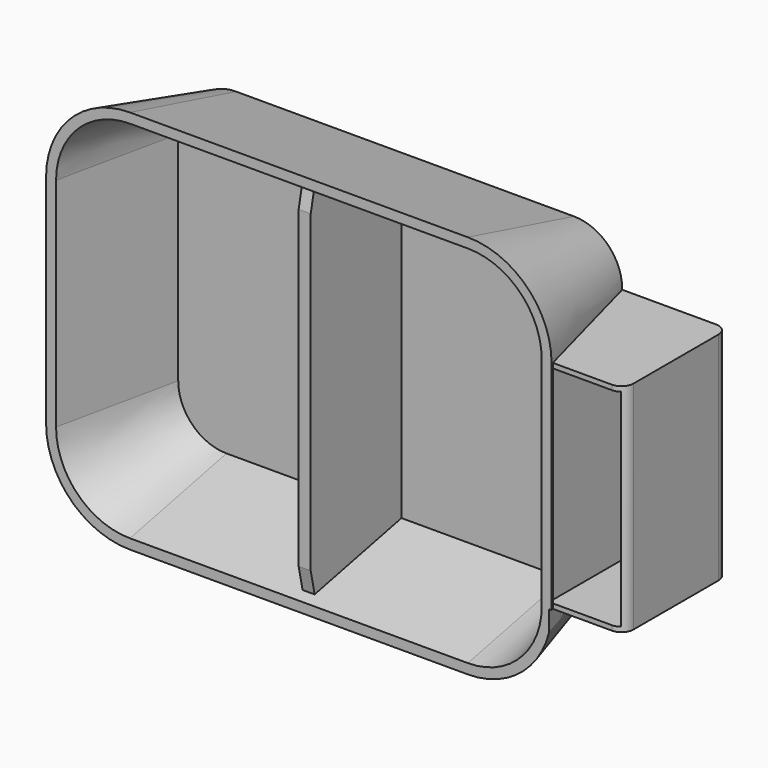
from build123d import *

# Parameters (mm, degrees)
F1_DEPTH     = 55
F1_TAPER     = -15
F4_DEPTH     = 55
F4_TAPER     = -12
F5_W         = 5
F5_H         = 130
F6_DEPTH     = 47
F10_W        = 360.01701653
F10_H        = 225.87454319
F11_DEPTH    = 25
F12_W        = 5
F12_H        = 46
F13_DEPTH    = 15
F14_W        = 5
F14_H        = 46
F15_DEPTH    = 15
F8_W         = 54.0339685977
F8_H         = 90.1
F16_DEPTH    = 32.6
F9_W         = 55.9400806222
F9_H         = 89.7377200425
F17_DEPTH    = 25
F18_W        = 347.7291613817
F18_H        = 217.2330617905
F19_DEPTH    = 25
F20_W        = 34.4053636551
F20_H        = 45.9854951713
F21_DEPTH    = 25
F22_W        = 1.5565819549
F22_H        = 85.7377200425
F22_W_2      = 27.4434180451
F23_DEPTH    = 52
F24_T1_DEPTH = 114.7377200425
F26_DEPTH    = 25
F27_W        = 5
F27_H        = 32
F28_DEPTH    = 10
F29_W        = 5
F29_H        = 35
F30_DEPTH    = 8
F31_W        = 122.5292943418
F31_H        = 48.8124843687
F32_DEPTH    = 25
F33_W        = 5
F33_H        = 6
F33_W_2      = 6
F34_DEPTH    = 32


# Not quite as in the source:
# - a fillet or chamfer that OpenCascade refuses, or shapes differently, is made with other operations: its cross-section is extruded or revolved along the edge and cut away or added
# - ends of sketch curves that miss each other by under 0.0002 mm in the source are joined


with BuildPart() as f1:
    # F0 (on Front) → F1 (new body)
    with BuildSketch(Plane.XZ):
        with BuildLine():
            Line((34.0782237053, 85.1892769337), (-105.9217762947, 85.1892769337))
            ThreePointArc((-105.9217762947, 85.1892769337), (-120.0639119184, 79.3314125574), (-125.9217762947, 65.1892769337))
            Line((-125.9217762947, 65.1892769337), (-125.9217762947, -24.8107230663))
            ThreePointArc((-125.9217762947, -24.8107230663), (-120.0639119184, -38.9528586901), (-105.9217762947, -44.8107230663))
            Line((-105.9217762947, -44.8107230663), (34.0782237053, -44.8107230663))
            ThreePointArc((34.0782237053, -44.8107230663), (48.220359329, -38.9528586901), (54.0782237053, -24.8107230663))
            Line((54.0782237053, -24.8107230663), (54.0782237053, 65.1892769337))
            ThreePointArc((54.0782237053, 65.1892769337), (48.220359329, 79.3314125574), (34.0782237053, 85.1892769337))
        make_face()
    extrude(amount=F1_DEPTH, taper=F1_TAPER)

    # F3 (on offset) → F4 (cut)
    with BuildSketch(Plane.XZ.offset(5)):
        with BuildLine():
            Line((34.106137666, 85.2195297501), (-105.893862334, 85.2195297501))
            ThreePointArc((-105.893862334, 85.2195297501), (-120.0359979577, 79.3616653739), (-125.893862334, 65.2195297501))
            Line((-125.893862334, 65.2195297501), (-125.893862334, -24.7804702499))
            ThreePointArc((-125.893862334, -24.7804702499), (-120.0359979577, -38.9226058736), (-105.893862334, -44.7804702499))
            Line((-105.893862334, -44.7804702499), (34.106137666, -44.7804702499))
            ThreePointArc((34.106137666, -44.7804702499), (48.2482732898, -38.9226058736), (54.106137666, -24.7804702499))
            Line((54.106137666, -24.7804702499), (54.106137666, 65.2195297501))
            ThreePointArc((54.106137666, 65.2195297501), (48.2482732898, 79.3616653739), (34.106137666, 85.2195297501))
        make_face()
    extrude(amount=F4_DEPTH, taper=F4_TAPER, mode=Mode.SUBTRACT)

    # F5 (on face) → F6 (join)
    with BuildSketch(Plane.XZ.offset(5)):
        with Locations((-35.893862334, 20.2195297501)):
            Rectangle(F5_W, F5_H)
    extrude(amount=F6_DEPTH)

    # F10 (on Front) → F11 (cut)
    with BuildSketch(Plane.XZ):
        with Locations((5.3876563907, 10.9746605158)):
            Rectangle(F10_W, F10_H)
    extrude(amount=-F11_DEPTH, mode=Mode.SUBTRACT)

    # F12 (on face) → F13 (join)
    with BuildSketch(Plane(origin=(0, 8.8907927165, -41.8278911112), x_dir=(1, 0, 0), z_dir=(0, -0.2079116908, 0.9781476007))):
        with Locations((-35.893862334, -37.2011212889)):
            Rectangle(F12_W, F12_H)
    extrude(amount=F13_DEPTH)

    # F14 (on face) → F15 (join)
    with BuildSketch(Plane(origin=(0, 17.1148163716, 80.5188804202), x_dir=(1, 0, 0), z_dir=(0, -0.2079116908, -0.9781476007))):
        with Locations((-35.893862334, 45.6088745247)):
            Rectangle(F14_W, F14_H)
    extrude(amount=F15_DEPTH)

    # F8 (on offset) → F16 (join)
    with BuildSketch(Plane.YZ.offset(98)):
        with Locations((-27.0169842988, 19.8769969761)):
            Rectangle(F8_W, F8_H)
    extrude(amount=-F16_DEPTH)

    # F9 (on face) → F17 (join)
    with BuildSketch(Plane(origin=(50.4556696128, 13.5195559263, 0), x_dir=(-0.2588190451, 0.9659258263, 0), z_dir=(0.9659258263, 0.2588190451, 0))):
        with Locations((-41.9665145313, 20.0581369549)):
            Rectangle(F9_W, F9_H)
    extrude(amount=F17_DEPTH)

    # F18 (on Front) → F19 (cut)
    with BuildSketch(Plane.XZ):
        with Locations((0.111065805, 20.1892703772)):
            Rectangle(F18_W, F18_H)
    extrude(amount=-F19_DEPTH, mode=Mode.SUBTRACT)

    # F20 (on face) → F21 (cut)
    with BuildSketch(Plane(origin=(0, 0, -24.8107230663), x_dir=(1, 0, 0), z_dir=(0, 0, -1))):
        Polygon((68.0166854944, 55.7510983837), (65.4, 45.9854951713), (99.8053636551, 45.9854951713), (100.283839941, 55.7510983837), align=None)
        with Locations((82.6026818275, 22.9927475857)):
            Rectangle(F20_W, F20_H)
    extrude(amount=F21_DEPTH, mode=Mode.SUBTRACT)

    # F22 (on face) → F23 (cut)
    with BuildSketch(Plane.XZ.offset(54.0339685977)):
        with Locations((67.7782909774, 20.0581369549)):
            Rectangle(F22_W, F22_H)
        with Locations((82.2782909774, 20.0581369549)):
            Rectangle(F22_W_2, F22_H)
    extrude(amount=-F23_DEPTH, mode=Mode.SUBTRACT)

    # F24: fillet of radius 5 on 2 edges, made by hand

    # F24_s2 → F24_t1 (cut)
    with BuildSketch(Plane.XY.offset(-37.3107230663)):
        with BuildLine():
            ThreePointArc((98, -49.0339685977), (96.5355339059, -52.5695025036), (93, -54.0339685977))
            Line((93, -54.0339685977), (98, -54.0339685977))
            Line((98, -54.0339685977), (98, -49.0339685977))
        make_face()
        with BuildLine():
            ThreePointArc((93, 0), (96.5355339059, -1.4644660941), (98, -5))
            Line((98, -5), (98, 0))
            Line((98, 0), (93, 0))
        make_face()
    extrude(amount=F24_T1_DEPTH, mode=Mode.SUBTRACT)

    # F25 (on face) → F26 (cut)
    with BuildSketch(Plane.XZ.offset(52)):
        Polygon((-33.3938625455, 92.2565162182), (-38.3938625455, 92.2565162182), (-38.3938625455, -53.0670173466), (-33.393862334, -53.0670173466), align=None)
    extrude(amount=F26_DEPTH, mode=Mode.SUBTRACT)

    # F27 (on face) → F28 (cut)
    with BuildSketch(Plane(origin=(0, 0, 0), x_dir=(-1, 0, 0), z_dir=(0, 1, 0))):
        with Locations((-90.5, 45.9269969761)):
            Rectangle(F27_W, F27_H)
    extrude(amount=-F28_DEPTH, mode=Mode.SUBTRACT)

    # F29 (on face) → F30 (join)
    with BuildSketch(Plane(origin=(0, 11.2026807666, -41.8089738019), x_dir=(1, 0, 0), z_dir=(0, 0.2588190451, -0.9659258263))):
        with Locations((-63.4217762947, 29.0978685544)):
            Rectangle(F29_W, F29_H)
        with Locations((-8.4217762947, 29.0978685544)):
            Rectangle(F29_W, F29_H)
    extrude(amount=F30_DEPTH)

    # F31 (on face) → F32 (cut)
    with BuildSketch(Plane(origin=(0, 0, 0), x_dir=(-1, 0, 0), z_dir=(0, 1, 0))):
        with Locations((32.052250579, -48.6711980775)):
            Rectangle(F31_W, F31_H)
    extrude(amount=F32_DEPTH, mode=Mode.SUBTRACT)

    # F33 (on face) → F34 (cut)
    with BuildSketch(Plane(origin=(0, -45.0100846867, -12.0604158431), x_dir=(1, 0, 0), z_dir=(0, -0.9659258263, -0.2588190451))):
        with Locations((-63.4217762947, -46.2838347045)):
            Rectangle(F33_W, F33_H)
        with Locations((-8.7768949285, -46.2838347045)):
            Rectangle(F33_W_2, F33_H)
    extrude(amount=-F34_DEPTH, mode=Mode.SUBTRACT)


solid = f1.part
